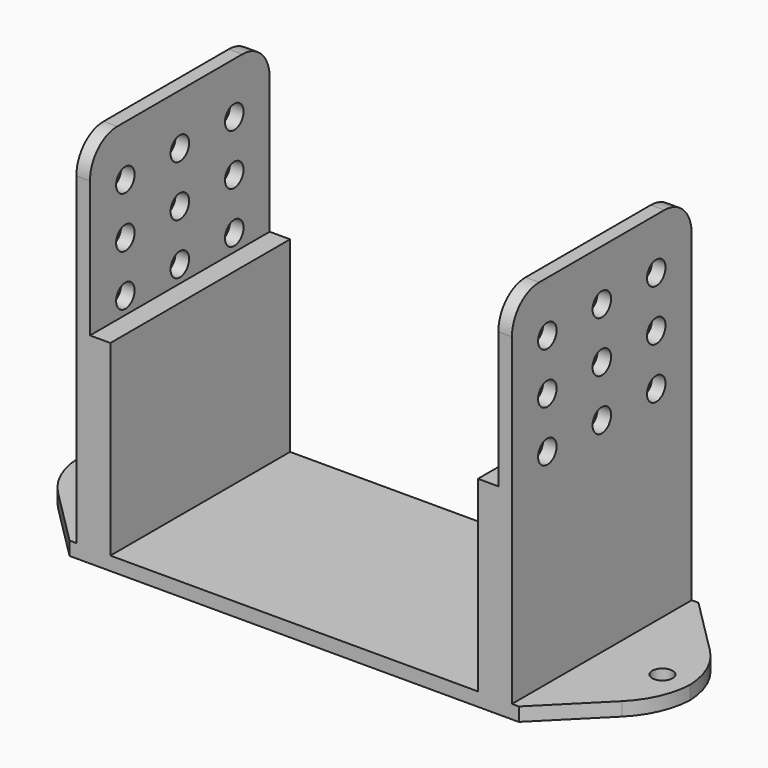
from build123d import *

# Parameters (mm, degrees)
F0_W         = 90
F0_H         = 33
F0_R         = 1.5
F1_DEPTH     = 2
F2_W         = 5
F2_H         = 33
F3_DEPTH     = 27.5
F4_W         = 2
F4_H         = 33
F5_DEPTH     = 25
F6_W         = 2
F6_H         = 33
F7_DEPTH     = 25
F9_D         = 3.4
F10_R        = 5
F11_SIZE     = 12
F12_T1_DEPTH = 27.1366974606


# Not quite as in the source:
# - a fillet or chamfer that OpenCascade refuses, or shapes differently, is made with other operations: its cross-section is extruded or revolved along the edge and cut away or added


with BuildPart() as f1:
    # F0 (on Top) → F1 (new body)
    with BuildSketch(Plane.XY):
        Rectangle(F0_W, F0_H)
        with Locations((-40.91, 0)):
            Circle(F0_R, mode=Mode.SUBTRACT)
        with Locations((40.91, 0)):
            Circle(F0_R, mode=Mode.SUBTRACT)
    extrude(amount=F1_DEPTH)

    # F2 (on face) → F3 (join)
    with BuildSketch(Plane.XY.offset(2)):
        with Locations((-29.5, 0)):
            Rectangle(F2_W, F2_H)
        with Locations((29.5, 0)):
            Rectangle(F2_W, F2_H)
    extrude(amount=F3_DEPTH)

    # F4 (on face) → F5 (join)
    with BuildSketch(Plane.XY.offset(29.5)):
        with Locations((-31, 0)):
            Rectangle(F4_W, F4_H)
    extrude(amount=F5_DEPTH)

    # F6 (on face) → F7 (join)
    with BuildSketch(Plane.XY.offset(29.5)):
        with Locations((31, 0)):
            Rectangle(F6_W, F6_H)
    extrude(amount=F7_DEPTH)

    # F9 (through all)
    with Locations(Plane(origin=(-32, 0, 0), x_dir=(0, -1, 0), z_dir=(-1, 0, 0))):
        with Locations((-10, 47), (-10, 39.5), (0, 39.5), (0, 47), (10, 47), (10, 39.5), (-10, 32), (0, 32), (10, 32)):
            Hole(F9_D / 2)

    # F10
    f10_edges = [f1.edges().sort_by_distance(p)[0] for p in [
        (-31, 16.5, 54.5),
        (31, 16.5, 54.5),
        (-31, -16.5, 54.5),
        (31, -16.5, 54.5),
    ]]
    fillet(f10_edges, radius=F10_R)

    # F11
    f11_edges = [f1.edges().sort_by_distance(p)[0] for p in [
        (45, 16.5, 1),
        (45, -16.5, 1),
        (-45, -16.5, 1),
        (-45, 16.5, 1),
    ]]
    chamfer(f11_edges, length=F11_SIZE)

    # F12: fillet of radius 12.1370711845 on 4 edges, made by hand

    # F12_s2 → F12_t1 (cut)
    with BuildSketch(Plane.XY.offset(-12.5683487303)):
        with BuildLine():
            ThreePointArc((41.4451341538, -8.0548658462), (44.0761204675, -4.1173165676), (45, 0.5273394921))
            Line((45, 0.5273394921), (45, -4.5))
            Line((45, -4.5), (41.4451341538, -8.0548658462))
        make_face()
        with BuildLine():
            ThreePointArc((45, -0.5273394921), (44.0761204675, 4.1173165676), (41.4451341538, 8.0548658462))
            Line((41.4451341538, 8.0548658462), (45, 4.5))
            Line((45, 4.5), (45, -0.5273394921))
        make_face()
        with BuildLine():
            ThreePointArc((-41.4451341538, -8.0548658462), (-44.0761204675, -4.1173165676), (-45, 0.5273394921))
            Line((-45, 0.5273394921), (-45, -4.5))
            Line((-45, -4.5), (-41.4451341538, -8.0548658462))
        make_face()
        with BuildLine():
            ThreePointArc((-45, -0.5273394921), (-44.0761204675, 4.1173165676), (-41.4451341538, 8.0548658462))
            Line((-41.4451341538, 8.0548658462), (-45, 4.5))
            Line((-45, 4.5), (-45, -0.5273394921))
        make_face()
    extrude(amount=F12_T1_DEPTH, mode=Mode.SUBTRACT)


solid = f1.part
